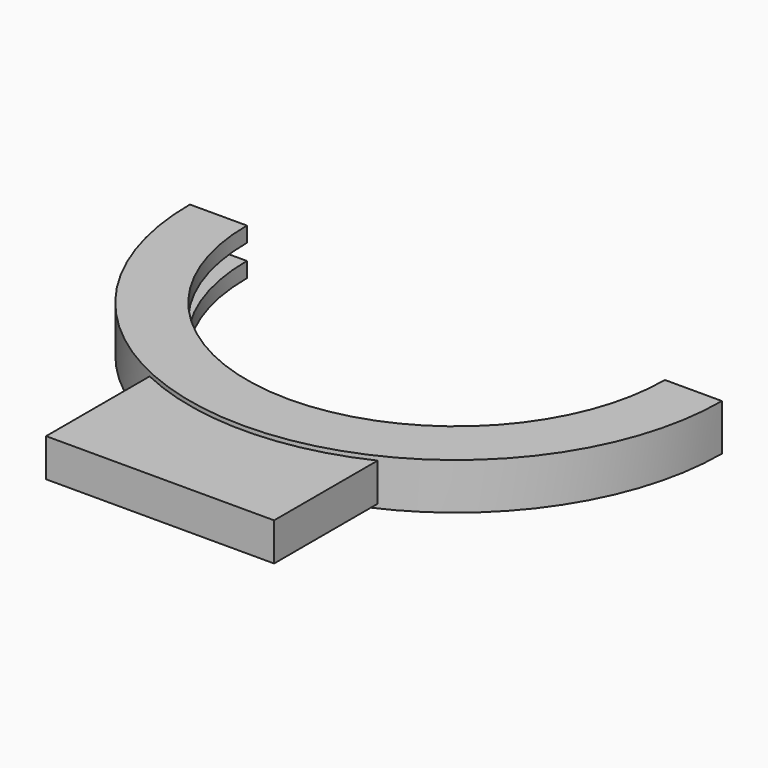
from build123d import *

# Parameters (mm, degrees)
F1_DEPTH = 1.05
F3_DEPTH = 2
F5_DEPTH = 2
F7_DEPTH = 2.5


with BuildPart() as f1:
    # F0 (on Top) → F1 (new body, symmetric)
    with BuildSketch(Plane.XY):
        with BuildLine():
            Line((35, 0), (30, 0))
            ThreePointArc((30, 0), (0, -30), (-30, 0))
            Line((-30, 0), (-35, 0))
            ThreePointArc((-35, 0), (0, -35), (35, 0))
        make_face()
    extrude(amount=F1_DEPTH, both=True)

    # F2 (on face) → F3 (join)
    with BuildSketch(Plane.XY.offset(1.05)):
        with BuildLine():
            ThreePointArc((-30, 0), (0, -30), (30, 0))
            Line((30, 0), (27.5, 0))
            ThreePointArc((27.5, 0), (0, -27.5), (-27.5, 0))
            Line((-27.5, 0), (-30, 0))
        make_face()
        with BuildLine():
            ThreePointArc((-35, 0), (0, -35), (35, 0))
            Line((35, 0), (30, 0))
            ThreePointArc((30, 0), (0, -30), (-30, 0))
            Line((-30, 0), (-35, 0))
        make_face()
    extrude(amount=F3_DEPTH)

    # F4 (on face) → F5 (join)
    with BuildSketch(Plane(origin=(0, 0, -1.05), x_dir=(1, 0, 0), z_dir=(0, 0, -1))):
        with BuildLine():
            Line((30, 0), (35, 0))
            ThreePointArc((35, 0), (0, 35), (-35, 0))
            Line((-35, 0), (-30, 0))
            ThreePointArc((-30, 0), (0, 30), (30, 0))
        make_face()
        with BuildLine():
            Line((27.5, 0), (30, 0))
            ThreePointArc((30, 0), (0, 30), (-30, 0))
            Line((-30, 0), (-27.5, 0))
            ThreePointArc((-27.5, 0), (0, 27.5), (27.5, 0))
        make_face()
    extrude(amount=F5_DEPTH)

    # F6 (on Top) → F7 (join, symmetric)
    with BuildSketch(Plane.XY):
        with BuildLine():
            Line((0, -48.6514897645), (0, -33.6514897645))
            ThreePointArc((0, -33.6514897645), (-7.624504365, -32.7740115893), (-15, -30.6514897645))
            Line((-15, -30.6514897645), (-15, -48.6514897645))
            Line((-15, -48.6514897645), (0, -48.6514897645))
        make_face()
        with BuildLine():
            ThreePointArc((15, -30.6514897645), (7.624504365, -32.7740115893), (0, -33.6514897645))
            Line((0, -33.6514897645), (0, -48.6514897645))
            Line((0, -48.6514897645), (15, -48.6514897645))
            Line((15, -48.6514897645), (15, -30.6514897645))
        make_face()
    extrude(amount=F7_DEPTH, both=True)


solid = f1.part
